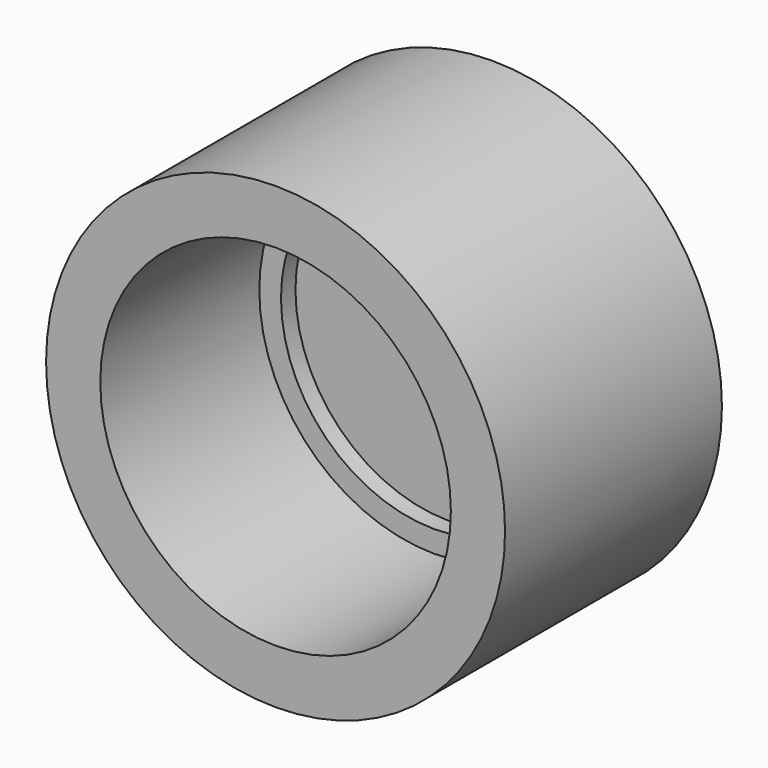
from build123d import *

# Parameters (mm, degrees)
F0_R          = 12.7
F0_R_2        = 9.7
F1_DEPTH      = 12
F1_DEPTH_BACK = 3
F0_R_3        = 8.5
F2_DEPTH      = 1
F3_DEPTH      = 3


with BuildPart() as f1:
    # F0 (on Front) → F1 (new body, two sides)
    with BuildSketch(Plane.XZ) as f1_sk:
        Circle(F0_R)
        Circle(F0_R_2, mode=Mode.SUBTRACT)
    extrude(amount=F1_DEPTH)
    extrude(f1_sk.sketch, amount=-F1_DEPTH_BACK)

    # F0 (on Front) → F3 (join)
    with BuildSketch(Plane.XZ):
        Circle(F0_R)
        Circle(F0_R_2, mode=Mode.SUBTRACT)
        Circle(F0_R_2)
        Circle(F0_R_3, mode=Mode.SUBTRACT)
        Circle(F0_R_3)
    extrude(amount=-F3_DEPTH)


with BuildPart() as f2:
    # F0 (on Front) → F2 (new body)
    with BuildSketch(Plane.XZ):
        Circle(F0_R_2)
        Circle(F0_R_3, mode=Mode.SUBTRACT)
    extrude(amount=F2_DEPTH)


solid = Compound([f1.part, f2.part])
